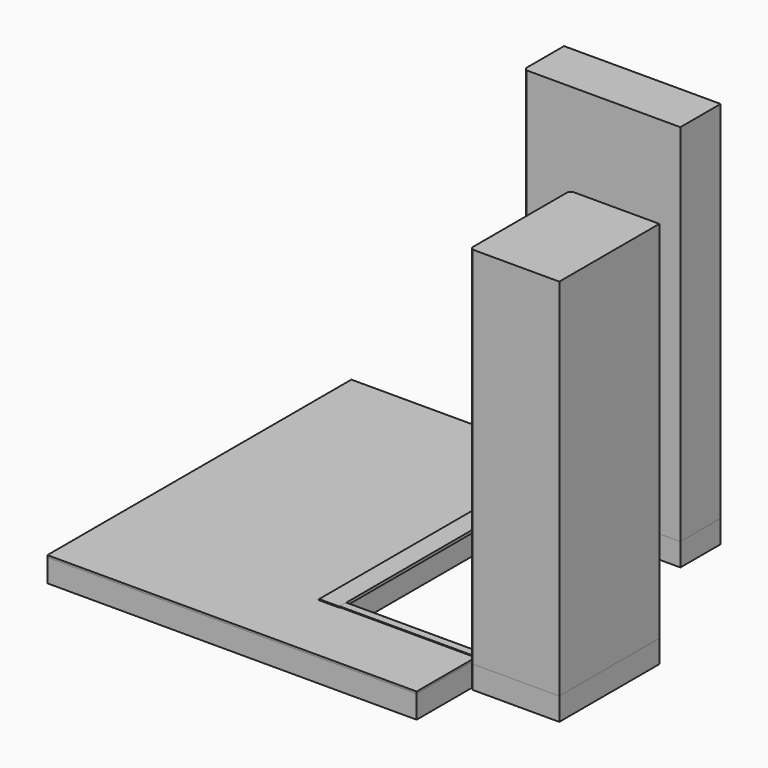
from build123d import *

# Parameters (mm, degrees)
F0_W      = 927.1
F0_H      = 336.3721848547
F0_H_2    = 533.5778151453
F1_DEPTH  = 152.4
F3_DEPTH  = 2438.4
F5_DEPTH  = 152.4
F6_DEPTH  = 2438.4
F7_W      = 19.05
F7_H      = 1670.05
F8_DEPTH  = 19.05
F10_DEPTH = 2.286
F11_DEPTH = 11.43
F13_DEPTH = 908.05
F15_DEPTH = 2052.8028121924
F16_W     = 17.9605122421
F16_H     = 13.716
F17_DEPTH = 2052.8028121924
F19_DEPTH = 1559.9841734515
F20_W     = 8.7408832695
F20_H     = 13.716
F21_DEPTH = 1559.9841734515


with BuildPart() as f1:
    # F0 (on Top) → F1 (new body)
    with BuildSketch(Plane.XY):
        Polygon((702.067170443, 931.1973798752), (702.067170443, 1267.5695647299), (-838.8660030085, 1267.5695647299), (-838.8660030085, -1272.4304352701), (702.067170443, -1272.4304352701), (702.067170443, -738.8526201248), align=None)
        with Locations((1165.617170443, 1099.3834723026)):
            Rectangle(F0_W, F0_H)
        with Locations((1165.617170443, -1005.6415276974)):
            Rectangle(F0_W, F0_H_2)
    extrude(amount=-F1_DEPTH)

    # F4 (on face) → F5 (join, through all)
    with BuildSketch(Plane.XY):
        Polygon((1629.167170443, -738.8526201248), (1629.167170443, -808.7026201248), (1647.1276826851, -826.663132367), (2226.1154003136, -826.663132367), (2226.1154003136, 9.3578921173), (1647.1276826851, 9.3578921173), (1629.167170443, -8.6026201248), align=None)
    extrude(amount=-F5_DEPTH)


with BuildPart() as f3:
    # F2 (on face) → F3 (new body)
    with BuildSketch(Plane.XY):
        Polygon((600.467170443, 931.1973798752), (702.067170443, 931.1973798752), (1629.167170443, 931.1973798752), (1629.167170443, 1267.5695647299), (582.5066582008, 1267.5695647299), (582.5066582008, 949.1578921173), align=None)
    extrude(amount=F3_DEPTH)


with BuildPart() as f6:
    # F4 (on face) → F6 (new body, through all)
    with BuildSketch(Plane.XY):
        Polygon((1629.167170443, -738.8526201248), (1629.167170443, -808.7026201248), (1647.1276826851, -826.663132367), (2226.1154003136, -826.663132367), (2226.1154003136, 9.3578921173), (1647.1276826851, 9.3578921173), (1629.167170443, -8.6026201248), align=None)
    extrude(amount=F6_DEPTH)


with BuildPart() as f8:
    # F7 (on face) → F8 (new body)
    with BuildSketch(Plane.XY):
        Polygon((702.067170443, 931.1973798752), (600.467170443, 931.1973798752), (582.5066582008, 949.1578921173), (582.5066582008, -785.2322474625), (721.117170443, -785.2322474625), (721.117170443, -738.8526201248), (702.067170443, -738.8526201248), align=None)
        with Locations((711.592170443, 96.1723798752)):
            Rectangle(F7_W, F7_H)
    extrude(amount=F8_DEPTH)

    # F14 (on face) → F15 (cut, through all)
    with BuildSketch(Plane.XZ.offset(785.2322474625)):
        Polygon((582.5066582008, 15.875), (585.6816582008, 19.05), (582.5066582008, 19.05), align=None)
    extrude(amount=-F15_DEPTH, mode=Mode.SUBTRACT)

    # F16 (on face) → F17 (cut, through all)
    with BuildSketch(Plane.XZ.offset(785.2322474625)):
        with Locations((591.4869143219, 6.858)):
            Rectangle(F16_W, F16_H)
    extrude(amount=-F17_DEPTH, mode=Mode.SUBTRACT)

    # F18 (on face) → F19 (cut, through all)
    with BuildSketch(Plane.YZ.offset(721.117170443)):
        Polygon((-782.0572474625, 19.05), (-785.2322474625, 19.05), (-785.2322474625, 15.875), align=None)
    extrude(amount=-F19_DEPTH, mode=Mode.SUBTRACT)

    # F20 (on face) → F21 (cut, through all)
    with BuildSketch(Plane.YZ.offset(721.117170443)):
        with Locations((-780.8618058277, 6.858)):
            Rectangle(F20_W, F20_H)
    extrude(amount=-F21_DEPTH, mode=Mode.SUBTRACT)


with BuildPart() as f10:
    # F9 (on face) → F10 (new body)
    with BuildSketch(Plane.XY):
        Polygon((582.5066582008, 949.1578921173), (582.5066582008, 1267.5695647299), (-838.8660030085, 1267.5695647299), (-838.8660030085, -1272.4304352701), (1629.167170443, -1272.4304352701), (1629.167170443, -808.7026201248), (1629.167170443, -779.666364193), (597.292170443, -779.666364193), (597.292170443, 934.3723798752), align=None)
    extrude(amount=F10_DEPTH)


with BuildPart() as f11:
    # F11 (new): a face of the model
    f11_faces = [f10.part.faces().sort_by_distance(p)[0] for p in [
        (29.5294646576, -129.086705172, 2.286),
    ]]
    extrude(f11_faces, amount=F11_DEPTH)


with BuildPart() as f13:
    # F12 (on face) → F13 (new body, through all)
    with BuildSketch(Plane.YZ.offset(721.117170443)):
        with BuildLine():
            Line((-762.9826201248, 0), (-738.8526201248, 0))
            Line((-738.8526201248, 0), (-721.2888350697, 0))
            ThreePointArc((-721.2888350697, 0), (-718.2244131725, 10.8423506116), (-725.9433340729, 19.05))
            Line((-725.9433340729, 19.05), (-779.7466201248, 19.05))
            ThreePointArc((-779.7466201248, 19.05), (-780.6322757019, 16.2147814743), (-778.2226201248, 14.478))
            Line((-778.2226201248, 14.478), (-762.9826201248, 14.478))
            Line((-762.9826201248, 14.478), (-762.9826201248, 0))
        make_face()
        with BuildLine():
            Line((-779.7466201248, 19.05), (-725.9433340729, 19.05))
            ThreePointArc((-725.9433340729, 19.05), (-727.8044343417, 19.4614100495), (-729.7080159187, 19.558))
            Line((-729.7080159187, 19.558), (-778.2226201248, 19.558))
            ThreePointArc((-778.2226201248, 19.558), (-779.0258386505, 19.427655577), (-779.7466201248, 19.05))
        make_face()
    extrude(amount=F13_DEPTH)


solid = Compound([f1.part, f3.part, f6.part, f8.part, f10.part, f11.part, f13.part])
